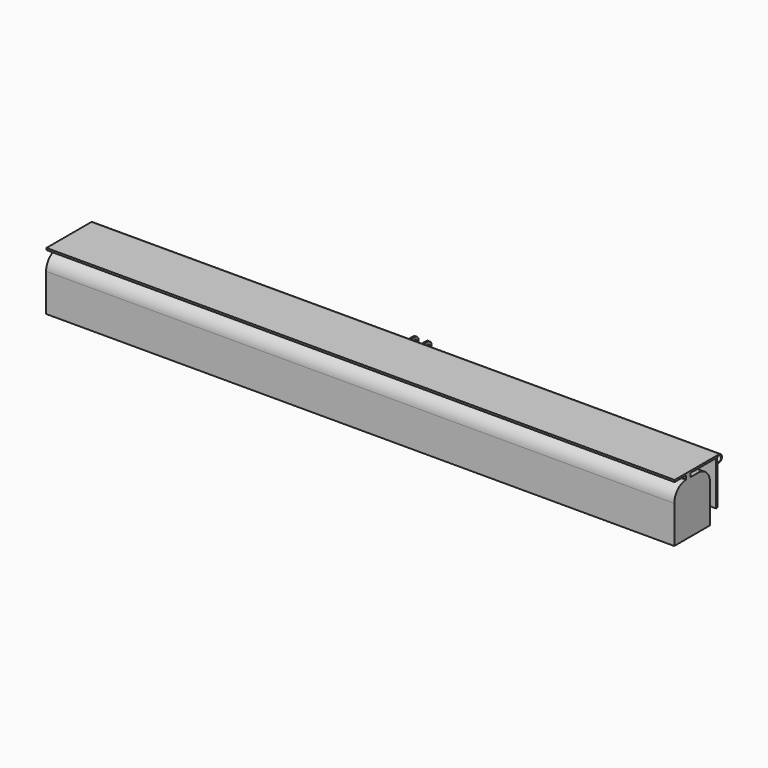
from build123d import *

# Parameters (mm, degrees)
F0_R          = 4.7625
F1_DEPTH      = 1079.5
F3_R          = 3.937
F4_DEPTH      = 12.7
F4_DEPTH_BACK = 12.7
F5_W          = 19.05
F5_H          = 60.4399840052
F6_DEPTH      = 84.921


# Not quite as in the source:
# - a feature names something its author has since deleted; it is built from what else it names


with BuildPart() as f1:
    # F0 (on Right) → F1 (new body)
    with BuildSketch(Plane.YZ):
        with BuildLine():
            Line((-11.938, 0), (0, 0))
            Line((0, 0), (0, -3.048))
            Line((0, -3.048), (0, -8.6186548987))
            Line((0, -8.6186548987), (0, -75.9830698371))
            Line((0, -75.9830698371), (3.302, -75.9830698371))
            Line((3.302, -75.9830698371), (3.302, -8.6186548987))
            ThreePointArc((3.302, -8.6186548987), (12.5020792667, -4.6210291468), (6.35, 3.302))
            Line((6.35, 3.302), (-88.9, 3.302))
            Line((-88.9, 3.302), (-88.9, 0))
            Line((-88.9, 0), (-76.962, 0))
            Line((-76.962, 0), (-64.3, 0))
            Line((-64.3, 0), (-64.3, -6.35))
            ThreePointArc((-64.3, -6.35), (-82.2605122421, -13.7894877579), (-89.7, -31.75))
            Line((-89.7, -31.75), (-89.7, -96.35))
            Line((-89.7, -96.35), (-12.7, -96.35))
            Line((-12.7, -96.35), (-12.7, -31.75))
            ThreePointArc((-12.7, -31.75), (-20.1394877579, -13.7894877579), (-38.1, -6.35))
            Line((-38.1, -6.35), (-54.3371811509, -6.35))
            Line((-54.3371811509, -6.35), (-54.3371811509, 0))
            Line((-54.3371811509, 0), (-11.938, 0))
        make_face()
        with Locations((6.35, -3.048)):
            Circle(F0_R, mode=Mode.SUBTRACT)
    extrude(amount=F1_DEPTH)

    # F3 (on offset) → F4 (join, two sides)
    with BuildSketch(Plane.YZ.offset(539.75)) as f4_sk:
        with BuildLine():
            Line((3.302, -11.43), (3.302, -68.58))
            Line((3.302, -68.58), (17.5895, -68.58))
            Line((17.5895, -68.58), (46.489693531, -23.6623454656))
            ThreePointArc((46.489693531, -23.6623454656), (46.7820764127, -15.5652920647), (39.8145, -11.43))
            Line((39.8145, -11.43), (3.302, -11.43))
        make_face()
        with Locations((39.8145, -19.3675)):
            Circle(F3_R, mode=Mode.SUBTRACT)
    extrude(amount=F4_DEPTH)
    extrude(f4_sk.sketch, amount=-F4_DEPTH_BACK)

    # F5 (on face) → F6 (cut, through all)
    with BuildSketch(Plane.XY.offset(-11.43)):
        with Locations((539.75, 36.6969920026)):
            Rectangle(F5_W, F5_H)
    extrude(amount=-F6_DEPTH, mode=Mode.SUBTRACT)


solid = f1.part
